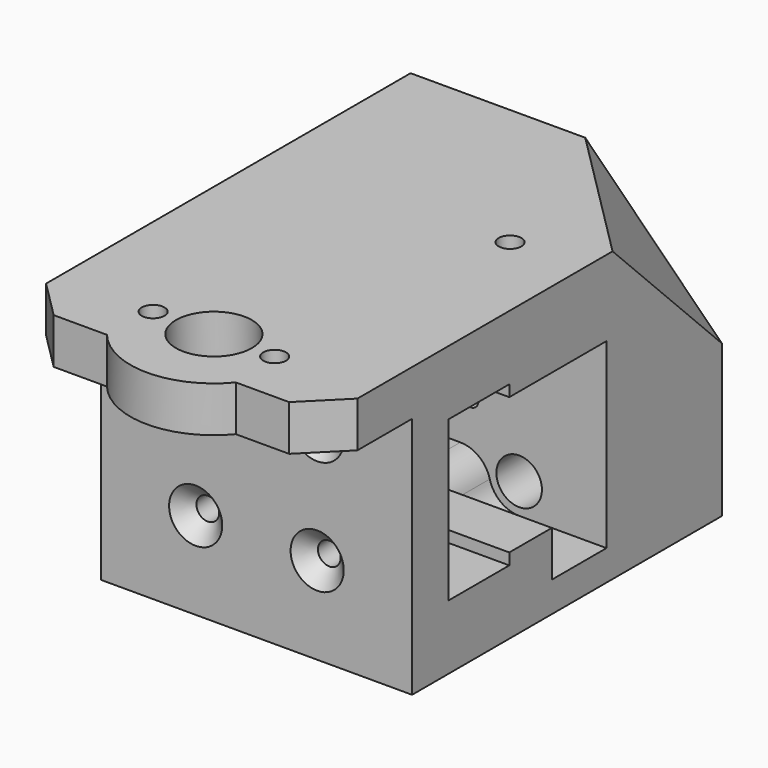
from build123d import *

# Parameters (mm, degrees)
F1_DEPTH  = 20.5
F2_R      = 1.5
F2_R_2    = 5
F3_DEPTH  = 6.001
F5_DEPTH  = 6
F6_R      = 1.5
F7_DEPTH  = 24.001
F8_SIZE   = 2
F9_R      = 1.5
F10_DEPTH = 38.001
F11_W     = 41
F11_H     = 38
F11_R     = 3
F11_R_2   = 1
F12_DEPTH = 19
F13_R     = 3
F14_DEPTH = 28
F16_DEPTH = 28
F17_R     = 4
F18_DEPTH = 9
F19_W     = 18
F19_H     = 18
F20_DEPTH = 18
F21_SIZE  = 17.99999
F22_SIZE  = 5
F24_DEPTH = 9
F25_R     = 4


# Not quite as in the source:
# - a fillet or chamfer is up to 0.001 mm smaller than in the source, because OpenCascade refuses the exact size


with BuildPart() as f1:
    # F0 (on Right) → F1 (new body, symmetric)
    with BuildSketch(Plane.YZ):
        Polygon((0, -10.5), (0, 10.5), (10, 10.5), (10, 9), (26, 9), (26, 19), (-20, 19), (-20, 13), (-6, 13), (-6, -19), (26, -19), (26, -9), (10, -9), (10, -10.5), align=None)
    extrude(amount=F1_DEPTH, both=True)

    # F2 (on face) → F3 (cut, through all)
    with BuildSketch(Plane(origin=(0, 0, 13), x_dir=(1, 0, 0), z_dir=(0, 0, -1))):
        with Locations((-8, 13)):
            Circle(F2_R)
        with Locations((8, 13)):
            Circle(F2_R)
        with Locations((0, 13)):
            Circle(F2_R_2)
    extrude(amount=-F3_DEPTH, mode=Mode.SUBTRACT)

    # F4 (on face) → F5 (join, through all)
    with BuildSketch(Plane.XY.offset(19)):
        with BuildLine():
            ThreePointArc((-8.4852813742, -20), (0, -24), (8.4852813742, -20))
            Line((8.4852813742, -20), (-8.4852813742, -20))
        make_face()
    extrude(amount=-F5_DEPTH)

    # F6 (on face) → F7 (cut, through all)
    with BuildSketch(Plane(origin=(0, 0, 0), x_dir=(-1, 0, 0), z_dir=(0, 1, 0))):
        with Locations((-8, 7.5)):
            Circle(F6_R)
        with Locations((8, 7.5)):
            Circle(F6_R)
        with Locations((8, -7.5)):
            Circle(F6_R)
        with Locations((-8, -7.5)):
            Circle(F6_R)
    extrude(amount=-F7_DEPTH, mode=Mode.SUBTRACT)

    # F8
    f8_edges = [f1.edges().sort_by_distance(p)[0] for p in [
        (-6.5, -6, 7.5),
        (9.5, -6, 7.5),
        (9.5, -6, -7.5),
        (-6.5, -6, -7.5),
    ]]
    chamfer(f8_edges, length=F8_SIZE)

    # F9 (on face) → F10 (cut, through all)
    with BuildSketch(Plane.XY.offset(19)):
        with Locations((-11, 22)):
            Circle(F9_R)
        with Locations((11, 22)):
            Circle(F9_R)
    extrude(amount=-F10_DEPTH, mode=Mode.SUBTRACT)

    # F11 (on face) → F12 (join)
    with BuildSketch(Plane(origin=(0, 26, 0), x_dir=(-1, 0, 0), z_dir=(0, 1, 0))):
        Rectangle(F11_W, F11_H)
        with Locations((-9, -11)):
            Circle(F11_R, mode=Mode.SUBTRACT)
        with Locations((-2.625, -3.5)):
            Circle(F11_R_2, mode=Mode.SUBTRACT)
        with Locations((2.625, 3.5)):
            Circle(F11_R_2, mode=Mode.SUBTRACT)
        with Locations((9, 11)):
            Circle(F11_R, mode=Mode.SUBTRACT)
    extrude(amount=F12_DEPTH)

    # F13 (on face) → F14 (cut)
    with BuildSketch(Plane(origin=(0, 45, 0), x_dir=(-1, 0, 0), z_dir=(0, 1, 0))):
        with Locations((9, 11)):
            Circle(F13_R)
        with Locations((-9, -11)):
            Circle(F13_R)
    extrude(amount=-F14_DEPTH, mode=Mode.SUBTRACT)

    # F15 (on face) → F16 (join, through all)
    with BuildSketch(Plane(origin=(0, 17, 0), x_dir=(-1, 0, 0), z_dir=(0, 1, 0))):
        with BuildLine():
            ThreePointArc((6.7639320225, 9), (9, 14), (11.2360679775, 9))
            Line((11.2360679775, 9), (20.5, 9))
            Line((20.5, 9), (20.5, 19))
            Line((20.5, 19), (0, 19))
            Line((0, 19), (0, 9))
            Line((0, 9), (6.7639320225, 9))
        make_face()
        with BuildLine():
            ThreePointArc((-6.7639320225, -9), (-9, -14), (-11.2360679775, -9))
            Line((-11.2360679775, -9), (-20.5, -9))
            Line((-20.5, -9), (-20.5, -19))
            Line((-20.5, -19), (0, -19))
            Line((0, -19), (0, -9))
            Line((0, -9), (-6.7639320225, -9))
        make_face()
    extrude(amount=F16_DEPTH)

    # F17 (on face) → F18 (cut, through all)
    with BuildSketch(Plane(origin=(0, 17, 0), x_dir=(-1, 0, 0), z_dir=(0, 1, 0))):
        with Locations((9, 11)):
            Circle(F17_R)
        with Locations((-9, -11)):
            Circle(F17_R)
    extrude(amount=F18_DEPTH, mode=Mode.SUBTRACT)

    # F19 (on face) → F20 (cut)
    with BuildSketch(Plane(origin=(0, 45, 0), x_dir=(-1, 0, 0), z_dir=(0, 1, 0))):
        with Locations((-11.5, 10)):
            Rectangle(F19_W, F19_H)
        with Locations((11.5, -10)):
            Rectangle(F19_W, F19_H)
    extrude(amount=-F20_DEPTH, mode=Mode.SUBTRACT)

    # F21 (size 18 in the source; OpenCascade refuses exactly that, so slightly less here)
    f21_edges = [f1.edges().sort_by_distance(p)[0] for p in [
        (2.5, 27, 10),
        (-2.5, 27, -10),
        (11.5, 27, 1),
        (2.5, 36, 1),
        (-2.5, 36, -1),
        (-11.5, 27, -1),
    ]]
    chamfer(f21_edges, length=F21_SIZE)

    # F22
    f22_edges = [f1.edges().sort_by_distance(p)[0] for p in [
        (20.5, -20, 16),
        (-20.5, -20, 16),
    ]]
    chamfer(f22_edges, length=F22_SIZE)

    # F23 (on face) → F24 (cut, through all)
    with BuildSketch(Plane.XZ.offset(-26)):
        with BuildLine():
            Line((20.5, -9), (12.4641016151, -9))
            ThreePointArc((12.4641016151, -9), (12.4641016151, -13), (9, -15))
            Line((9, -15), (20.5, -15))
            Line((20.5, -15), (20.5, -9))
        make_face()
        with BuildLine():
            Line((-20.5, 9), (-12.4641016151, 9))
            ThreePointArc((-12.4641016151, 9), (-12.4641016151, 13), (-9, 15))
            Line((-9, 15), (-20.5, 15))
            Line((-20.5, 15), (-20.5, 9))
        make_face()
    extrude(amount=F24_DEPTH, mode=Mode.SUBTRACT)

    # F25
    f25_edges = [f1.edges().sort_by_distance(p)[0] for p in [
        (-5.535898, 21.5, 9),
        (5.535898, 21.5, -9),
    ]]
    fillet(f25_edges, radius=F25_R)


solid = f1.part
